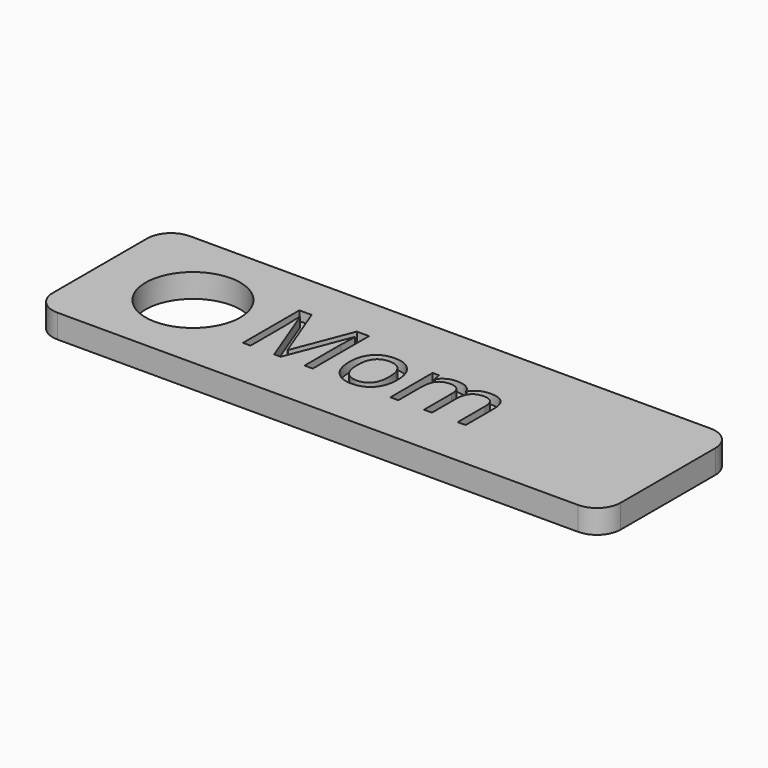
from build123d import *

# Parameters (mm, degrees)
F0_W         = 120
F0_H         = 35
F0_R         = 10
F1_DEPTH     = 5
F2_R         = 5
F3_TEXT_SIZE = 20.8333333333
F4_DEPTH     = 2


# Not quite as in the source:
# - Text() gives the source's letters only with a copy of the font that has no kerning and outlines rounded to 1/6400 em; it was checked with that copy


with BuildPart() as f1:
    # F0 (on Top) → F1 (new body)
    with BuildSketch(Plane.XY):
        Rectangle(F0_W, F0_H)
        with Locations((-40.3565168381, 0)):
            Circle(F0_R, mode=Mode.SUBTRACT)
    extrude(amount=F1_DEPTH)

    # F2
    f2_edges = [f1.edges().sort_by_distance(p)[0] for p in [
        (-60, -17.5, 2.5),
        (60, -17.5, 2.5),
        (60, 17.5, 2.5),
        (-60, 17.5, 2.5),
    ]]
    fillet(f2_edges, radius=F2_R)

    # F3 (on face) → F4 (cut)
    with BuildSketch(Plane.XY.offset(5)):
        with Locations((-26.3963251957, -6.7955985962)):
            Text('Mom', F3_TEXT_SIZE, font='Open Sans', text_align=(TextAlign.LEFT, TextAlign.BOTTOM))
    extrude(amount=-F4_DEPTH, mode=Mode.SUBTRACT)


solid = f1.part
